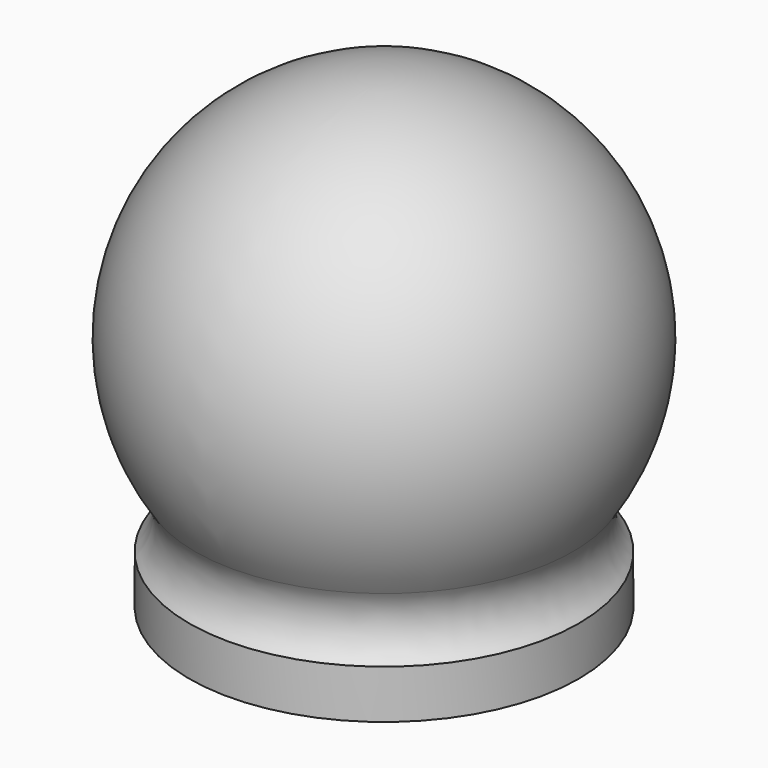
from build123d import *

# Parameters (mm, degrees)
F0_R     = 20
F1_DEPTH = 5
F5_T     = -2.5


# Not quite as in the source:
# - a fillet or chamfer that OpenCascade refuses, or shapes differently, is made with other operations: its cross-section is extruded or revolved along the edge and cut away or added


with BuildPart() as f1:
    # F0 (on Top) → F1 (new body)
    with BuildSketch(Plane.XY):
        Circle(F0_R)
    extrude(amount=F1_DEPTH)

    # F2 (on Right) → F3 (revolve)
    with BuildSketch(Plane.YZ):
        with BuildLine():
            Line((0, 0.953980596), (0, 47.7081678201))
            ThreePointArc((0, 47.7081678201), (-23.377093612, 24.331074208), (0, 0.953980596))
        make_face()
    revolve(axis=Axis((0, 0, 23.85408391), (0, 0, 1)))

    # F4: fillet of radius 5 on 1 edges, made by hand

    # F4_s1 → F4_t2 (revolve)
    with BuildSketch(Plane.YZ):
        with BuildLine():
            ThreePointArc((-20, 5), (-18.5807849657, 8.0440971034), (-19.4078057687, 11.2993597778))
            Line((-19.4078057687, 11.2993597778), (-19.3247851585, 11.3551054348))
            ThreePointArc((-19.3247851585, 11.3551054348), (-16.5075665861, 7.9200007382), (-13.0890367821, 5.0826923763))
            Line((-13.0890367821, 5.0826923763), (-13.1452681871, 4.9))
            ThreePointArc((-13.1452681871, 4.9), (-16.5726340935, 4.9), (-19.9288232744, 4.9297584615))
            Line((-19.9288232744, 4.9297584615), (-20, 5))
        make_face()
    revolve(axis=Axis((0, 0, 5), (0, 0, -1)))

    # F5
    f5_openings = [f1.faces().sort_by_distance(p)[0] for p in [
        (0, 0, 0),
    ]]
    offset(amount=F5_T, openings=f5_openings)


solid = f1.part
